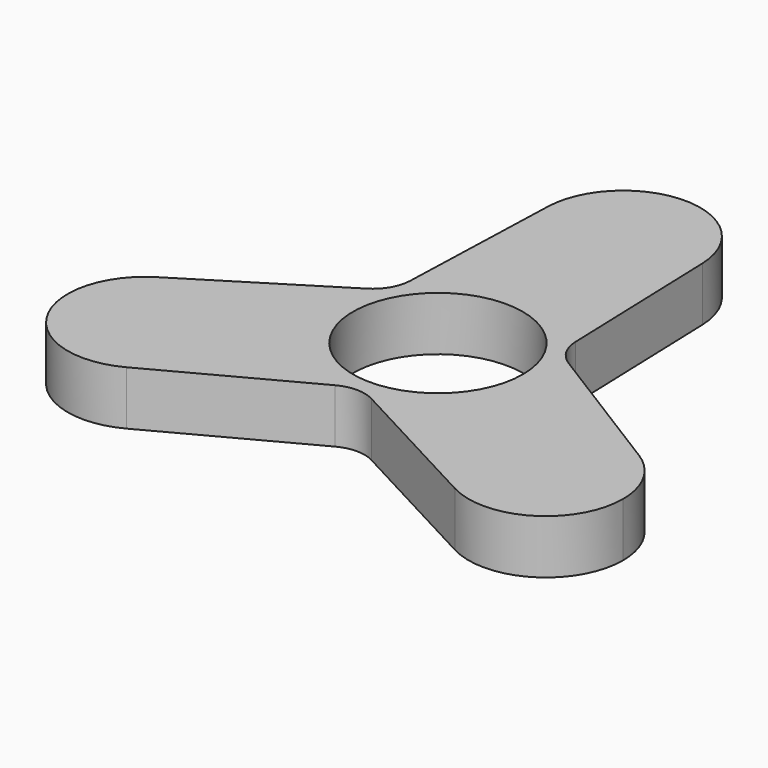
from build123d import *

# Parameters (mm, degrees)
F0_R     = 11
F1_DEPTH = 7
F3_R     = 8.5
F4_DEPTH = 4.2


# Not quite as in the source:
# - a feature names something its author has since deleted; it is built from what else it names


with BuildPart() as f1:
    # F0 (on Top) → F1 (new body)
    with BuildSketch(Plane.XY):
        with BuildLine():
            ThreePointArc((9.9944429004, 30.3333333333), (9.9986106286, 30.1666898261), (10, 30))
            ThreePointArc((10, 30), (-0.1666898261, 20.0013893714), (-9.9944429004, 30.3333333333))
            Line((-9.9944429004, 30.3333333333), (-10.7092358725, 8.9014606966))
            ThreePointArc((-10.7092358725, 8.9014606966), (-11.3763303038, 6.5681273633), (-13.0635090303, 4.8237399724))
            Line((-13.0635090303, 4.8237399724), (-31.2666586983, -6.5112252183))
            ThreePointArc((-31.2666586983, -6.5112252183), (-21.1258144232, -6.2576042801), (-15.9807621135, -15))
            ThreePointArc((-15.9807621135, -15), (-17.4050562197, -20.1436629382), (-21.2722157979, -23.8221081151))
            Line((-21.2722157979, -23.8221081151), (-2.3542731578, -13.725200669))
            ThreePointArc((-2.3542731578, -13.725200669), (0, -13.1362547266), (2.3542731578, -13.725200669))
            Line((2.3542731578, -13.725200669), (21.2722157979, -23.8221081151))
            ThreePointArc((21.2722157979, -23.8221081151), (17.3205080757, -10), (31.2666586983, -6.5112252183))
            Line((31.2666586983, -6.5112252183), (13.0635090303, 4.8237399724))
            ThreePointArc((13.0635090303, 4.8237399724), (11.3763303038, 6.5681273633), (10.7092358725, 8.9014606966))
            Line((10.7092358725, 8.9014606966), (9.9944429004, 30.3333333333))
        make_face()
        Circle(F0_R, mode=Mode.SUBTRACT)
        with BuildLine():
            ThreePointArc((-9.9944429004, 30.3333333333), (-0.1666898261, 20.0013893714), (10, 30))
            ThreePointArc((10, 30), (9.9986106286, 30.1666898261), (9.9944429004, 30.3333333333))
            ThreePointArc((9.9944429004, 30.3333333333), (0, 40), (-9.9944429004, 30.3333333333))
        make_face()
        with BuildLine():
            ThreePointArc((-15.9807621135, -15), (-21.1258144232, -6.2576042801), (-31.2666586983, -6.5112252183))
            ThreePointArc((-31.2666586983, -6.5112252183), (-34.6410161514, -20), (-21.2722157979, -23.8221081151))
            ThreePointArc((-21.2722157979, -23.8221081151), (-17.4050562197, -20.1436629382), (-15.9807621135, -15))
        make_face()
        with BuildLine():
            ThreePointArc((35.9807621135, -15), (34.7231578335, -10.1450523096), (31.2666586983, -6.5112252183))
            ThreePointArc((31.2666586983, -6.5112252183), (17.3205080757, -10), (21.2722157979, -23.8221081151))
            ThreePointArc((21.2722157979, -23.8221081151), (31.1244250518, -23.5757058939), (35.9807621135, -15))
        make_face()
    extrude(amount=F1_DEPTH)

    # F3 (on offset) → F4 (cut)
    with BuildSketch(Plane.XY.offset(1.4)):
        with Locations((25.9807621135, -15)):
            Circle(F3_R)
        with Locations((-25.9807621135, -15)):
            Circle(F3_R)
        with Locations((0, 30)):
            Circle(F3_R)
    extrude(amount=F4_DEPTH, mode=Mode.SUBTRACT)


solid = f1.part
